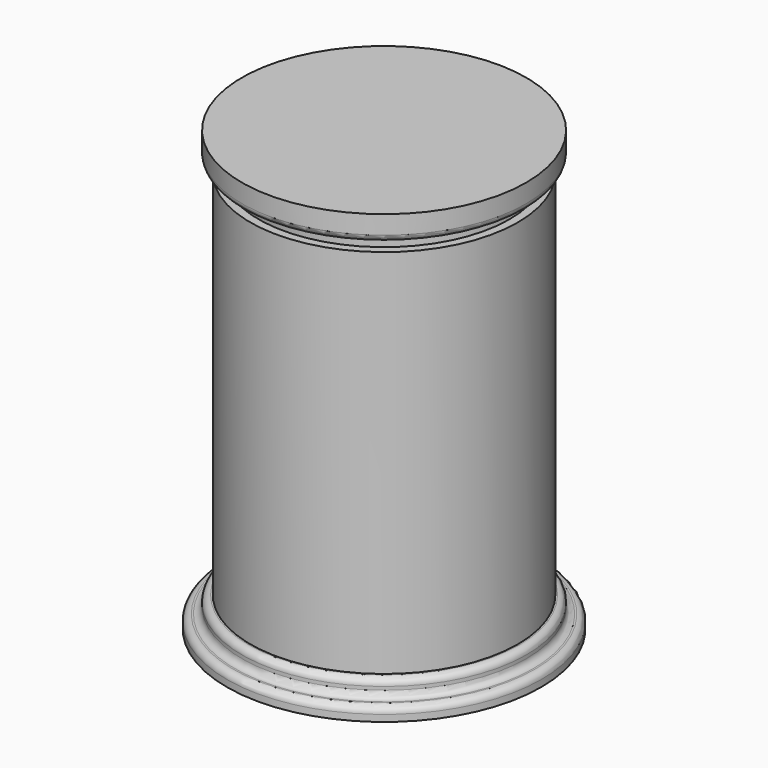
from build123d import *

# Parameters (mm, degrees)
F0_R     = 50.8
F0_R_2   = 47.625
F1_DEPTH = 152.4


# Not quite as in the source:
# - a fillet or chamfer that OpenCascade refuses, or shapes differently, is made with other operations: its cross-section is extruded or revolved along the edge and cut away or added


with BuildPart() as f1:
    # F0 (on Top) → F1 (new body)
    with BuildSketch(Plane.XY):
        Circle(F0_R)
        Circle(F0_R_2, mode=Mode.SUBTRACT)
    extrude(amount=F1_DEPTH)


with BuildPart() as f3:
    # F2 (on Front) → F3 (revolve)
    with BuildSketch(Plane.XZ):
        with BuildLine():
            Line((0, 6.35), (0, 0))
            Line((0, 0), (59.69, 0))
            Line((59.69, 0), (59.69, 2.54))
            ThreePointArc((59.69, 2.54), (58.9460512242, 4.3360512242), (57.15, 5.08))
            Line((57.15, 5.08), (56.515, 5.08))
            ThreePointArc((56.515, 5.08), (54.7189487758, 5.8239487758), (53.975, 7.62))
            Line((53.975, 7.62), (53.975, 8.89))
            ThreePointArc((53.975, 8.89), (53.2310512242, 10.6860512242), (51.435, 11.43))
            Line((51.435, 11.43), (50.8, 11.43))
            Line((50.8, 11.43), (50.8, 5.08))
            Line((50.8, 5.08), (44.45, 5.08))
            Line((44.45, 5.08), (44.45, 11.43))
            Line((44.45, 11.43), (38.1, 11.43))
            Line((38.1, 11.43), (38.1, 6.35))
            Line((38.1, 6.35), (0, 6.35))
        make_face()
    revolve(axis=Axis((0, 0, 3.175), (0, 0, -1)))


with BuildPart() as f5:
    # F4 (on Front) → F5 (revolve)
    with BuildSketch(Plane.XZ):
        Polygon((53.975, 166.7292495387), (0, 166.7292495387), (0, 164.8242495387), (52.07, 164.8242495387), (52.07, 157.24065432), (53.975, 157.24065432), align=None)
    revolve(axis=Axis((0, 0, 165.7767495387), (0, 0, 1)))

    # F6: fillet of radius 2.54 on 1 edges, made by hand

    # F6_s1 → F6_t2 (revolve, cut)
    with BuildSketch(Plane.XZ):
        with BuildLine():
            ThreePointArc((52.07, 157.24065432), (53.4430463142, 158.1445727582), (53.975, 159.6999987449))
            Line((53.975, 159.6999987449), (53.975, 157.24065432))
            Line((53.975, 157.24065432), (52.07, 157.24065432))
        make_face()
    revolve(axis=Axis((0, 0, 157.24065432), (0, 0, 1)), mode=Mode.SUBTRACT)


solid = Compound([f1.part, f3.part, f5.part])
